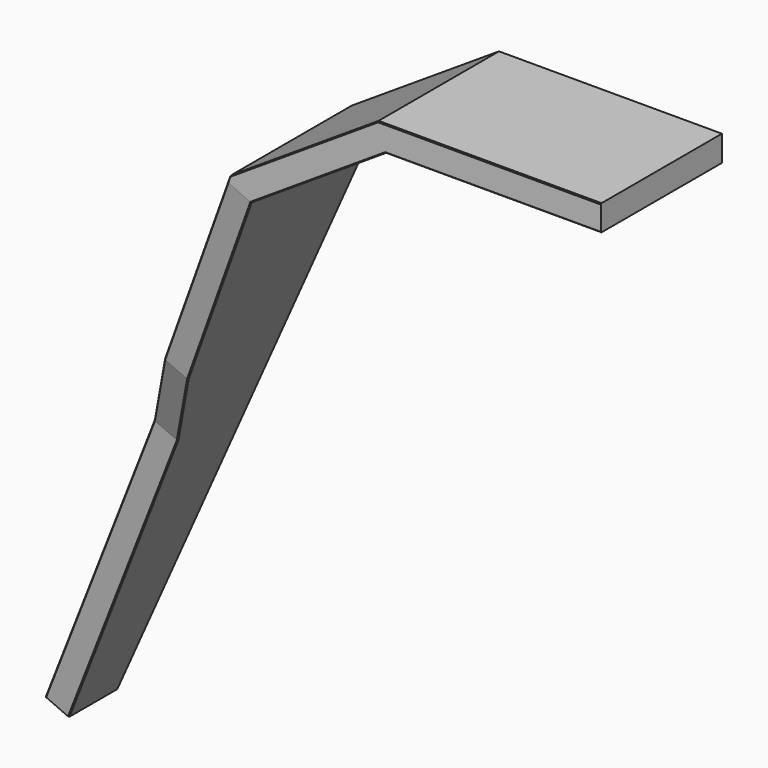
from build123d import *

# Parameters (mm, degrees)
F1_DEPTH     = 5
F3_DEPTH     = 25
F4_T1_DEPTH  = 5.9478639207
F4_T6_DEPTH  = 11.0004984696
F4_T11_DEPTH = 3.281815708
F4_T16_DEPTH = 7.2643009793
F4_T21_DEPTH = 5.7529029378
F5_T1_DEPTH  = 7.6329796459
F5_T3_DEPTH  = 7.4610000963
F5_T8_DEPTH  = 7.4842482227
F5_T13_DEPTH = 7.4842482227
F5_T18_DEPTH = 3.281815708
F5_T23_DEPTH = 11.0004984696


# Not quite as in the source:
# - a fillet or chamfer that OpenCascade refuses, or shapes differently, is made with other operations: its cross-section is extruded or revolved along the edge and cut away or added


with BuildPart() as f1:
    # F0 (on Front) → F1 (new body)
    with BuildSketch(Plane.XZ):
        Polygon((-7.11, 0), (0, 0), (0, 0.85), (-7.3617814707, 0.85), (-12.2206721932, -2.3054005297), (-20.7425294551, -21.4458053218), (-19.9660158161, -21.7915314684), (-11.5465673044, -2.8811404952), align=None)
    extrude(amount=F1_DEPTH)

    # F2 (on face) → F3 (cut)
    with BuildSketch(Plane(origin=(-8.5658121179, 0, 3.8137452678), x_dir=(0, 1, 0), z_dir=(0.9135454576, 0, -0.4067366431))):
        Polygon((-4, -14.4284648367), (-5, -7.3284648367), (-5, -28.0284648367), (-2, -28.0284648367), (-3, -17.2284648367), align=None)
    extrude(amount=-F3_DEPTH, mode=Mode.SUBTRACT)

    # F4: chamfer of 0.03 on 5 edges, made by hand

    # F4_s2 → F4_t1 (cut)
    with BuildSketch(Plane(origin=(-4.7250832121, 0, -3.0685049164), x_dir=(0, 1, 0), z_dir=(-0.8386705679, 0, -0.544639035))):
        Polygon((-4.97, -4.722383539), (-5, -4.692383539), (-5, -4.722383539), align=None)
    extrude(amount=F4_T1_DEPTH, mode=Mode.SUBTRACT)


with BuildPart() as f4_tool4:
    # F4_s5 → F4_t6 (new body)
    with BuildSketch(Plane(origin=(-11.2598610976, 2.5632795791, -25.2900620943), x_dir=(0.2219685938, 0.9750538156, 0), z_dir=(0.4050042191, -0.0921982106, 0.9096543698))):
        Polygon((-6.352559346, 8.2598889374), (-6.3880194376, 8.283182325), (-6.3819360855, 8.2538055854), align=None)
    extrude(amount=F4_T6_DEPTH)

    split(bisect_by=Plane(origin=(-0.3055183915, 0.3704168412, 0.2808368777), x_dir=(0.771450463, 0.6362893863, 0), z_dir=(0.549241742, -0.6659120918, -0.5048708694)), keep=Keep.TOP)


with BuildPart() as f1_1:
    add(f1.part)

    # F4_t3: cut F4_tool4
    add(f4_tool4.part, mode=Mode.SUBTRACT)


with BuildPart() as f4_tool9:
    # F4_s10 → F4_t11 (new body)
    with BuildSketch(Plane(origin=(-5.8578101844, 5.1435618144, -13.1568570886), x_dir=(0.659809773, 0.751432674, 0), z_dir=(0.3830409438, -0.336336397, 0.8603240456))):
        Polygon((-12.5057496784, 2.3040031535), (-12.5477702003, 2.3098577021), (-12.5296872137, 2.2859201669), align=None)
    extrude(amount=F4_T11_DEPTH)

    split(bisect_by=Plane(origin=(-2.1159962098, 2.405108563, 1.1858724964), x_dir=(0.7507908153, 0.6605400454, 0), z_dir=(0.6194574075, -0.7040949829, -0.3471639027)), keep=Keep.TOP)


with BuildPart() as f1_2:
    add(f1_1.part)

    # F4_t8: cut F4_tool9
    add(f4_tool9.part, mode=Mode.SUBTRACT)


with BuildPart() as f4_tool14:
    # F4_s15 → F4_t16 (new body)
    with BuildSketch(Plane.YZ.offset(-7.1871504896)):
        Polygon((-4.97, 0), (-5, 0.03), (-5, 0), align=None)
    extrude(amount=F4_T16_DEPTH)

    split(bisect_by=Plane(origin=(0.2989023851, -0.5488082305, -0.4602693104), x_dir=(0.878196468, 0.4783000769, 0), z_dir=(0.385117955, -0.7071067812, -0.5930296458)), keep=Keep.TOP)


with BuildPart() as f1_3:
    add(f1_2.part)

    # F4_t13: cut F4_tool14
    add(f4_tool14.part, mode=Mode.SUBTRACT)


with BuildPart() as f4_tool19:
    # F4_s20 → F4_t21 (new body)
    with BuildSketch(Plane(origin=(-9.7610352954, 0, -6.3388904383), x_dir=(0, 1, 0), z_dir=(0.8386705679, 0, 0.544639035))):
        Polygon((-4.97, 3.872383539), (-5, 3.902383539), (-5, 3.872383539), align=None)
    extrude(amount=F4_T21_DEPTH)

    split(bisect_by=Plane(origin=(-8.5658121179, 0, 3.8137452678), x_dir=(0, 1, 0), z_dir=(0.9135454576, 0, -0.4067366431)), keep=Keep.TOP)

    split(bisect_by=Plane(origin=(0, -2.485, -2.485), x_dir=(1, 0, 0), z_dir=(0, -0.7071067812, -0.7071067812)), keep=Keep.TOP)


with BuildPart() as f1_4:
    add(f1_3.part)

    # F4_t18: cut F4_tool19
    add(f4_tool19.part, mode=Mode.SUBTRACT)

    # F5: chamfer of 0.03 on 5 edges, made by hand

    # F5_s2 → F5_t1 (cut)
    with BuildSketch(Plane(origin=(-5.6229623165, 1.9471236166, -12.6293801411), x_dir=(0.3272176494, 0.9449489986, 0), z_dir=(0.4027614046, -0.1394685218, 0.9046169258))):
        Polygon((-8.7284463039, 7.9822536907), (-8.7481067262, 7.9446575766), (-8.7570745721, 7.9732858448), align=None)
    extrude(amount=F5_T1_DEPTH, mode=Mode.SUBTRACT)

    # F5_s4 → F5_t3 (cut)
    with BuildSketch(Plane.YZ.offset(-7.3838496067)):
        Polygon((-4.97, 0.85), (-5, 0.82), (-5, 0.85), align=None)
    extrude(amount=F5_T3_DEPTH, mode=Mode.SUBTRACT)


with BuildPart() as f5_tool6:
    # F5_s7 → F5_t8 (new body)
    with BuildSketch(Plane(origin=(-5.5630590396, 1.9263802648, -12.4948351783), x_dir=(0.3272176494, 0.9449489986, 0), z_dir=(0.4027614046, -0.1394685218, 0.9046169258))):
        Polygon((-8.4743573363, 7.1711194253), (-8.5119534504, 7.1907798476), (-8.5029856044, 7.1621515794), align=None)
    extrude(amount=F5_T8_DEPTH)

    split(bisect_by=Plane(origin=(0.2989023851, -0.5488082305, -0.4602693104), x_dir=(0.878196468, 0.4783000769, 0), z_dir=(0.385117955, -0.7071067812, -0.5930296458)), keep=Keep.TOP)


with BuildPart() as f1_5:
    add(f1_4.part)

    # F5_t5: cut F5_tool6
    add(f5_tool6.part, mode=Mode.SUBTRACT)


with BuildPart() as f5_tool11:
    # F5_s12 → F5_t13 (new body)
    with BuildSketch(Plane(origin=(-5.5630590396, 1.9263802648, -12.4948351783), x_dir=(0.3272176494, 0.9449489986, 0), z_dir=(0.4027614046, -0.1394685218, 0.9046169258))):
        Polygon((-8.4743573363, 7.1711194253), (-8.5119534504, 7.1907798476), (-8.5029856044, 7.1621515794), align=None)
    extrude(amount=F5_T13_DEPTH)

    split(bisect_by=Plane(origin=(-2.1090512339, 0, 3.2476541019), x_dir=(0, 1, 0), z_dir=(0.544639035, 0, -0.8386705679)), keep=Keep.TOP)


with BuildPart() as f1_6:
    add(f1_5.part)

    # F5_t10: cut F5_tool11
    add(f5_tool11.part, mode=Mode.SUBTRACT)


with BuildPart() as f5_tool16:
    # F5_s17 → F5_t18 (new body)
    with BuildSketch(Plane(origin=(-5.8578101844, 5.1435618144, -13.1568570886), x_dir=(0.659809773, 0.751432674, 0), z_dir=(0.3830409438, -0.336336397, 0.8603240456))):
        Polygon((-13.0181009663, 2.9822333193), (-13.0239555149, 2.9402127974), (-13.0420385015, 2.9641503327), align=None)
    extrude(amount=F5_T18_DEPTH)

    split(bisect_by=Plane(origin=(-7.0244742563, -7.3545925713, 2.3820711564), x_dir=(0.7231501661, -0.6906908406, 0), z_dir=(-0.6724909686, -0.7040949829, 0.2280485743)), keep=Keep.TOP)


with BuildPart() as f1_7:
    add(f1_6.part)

    # F5_t15: cut F5_tool16
    add(f5_tool16.part, mode=Mode.SUBTRACT)


with BuildPart() as f5_tool21:
    # F5_s22 → F5_t23 (new body)
    with BuildSketch(Plane(origin=(-11.2598610976, 2.5632795791, -25.2900620943), x_dir=(0.2219685938, 0.9750538156, 0), z_dir=(0.4050042191, -0.0921982106, 0.9096543698))):
        Polygon((-6.5249209865, 9.0922298921), (-6.548214374, 9.0567698005), (-6.554297726, 9.0861465401), align=None)
    extrude(amount=F5_T23_DEPTH)

    split(bisect_by=Plane(origin=(-9.881776244, -8.860018193, 0.9359011948), x_dir=(0.6675656779, -0.7445509155, 0), z_dir=(-0.742706634, -0.6659120918, 0.0703416075)), keep=Keep.TOP)


with BuildPart() as f1_8:
    add(f1_7.part)

    # F5_t20: cut F5_tool21
    add(f5_tool21.part, mode=Mode.SUBTRACT)


solid = f1_8.part
